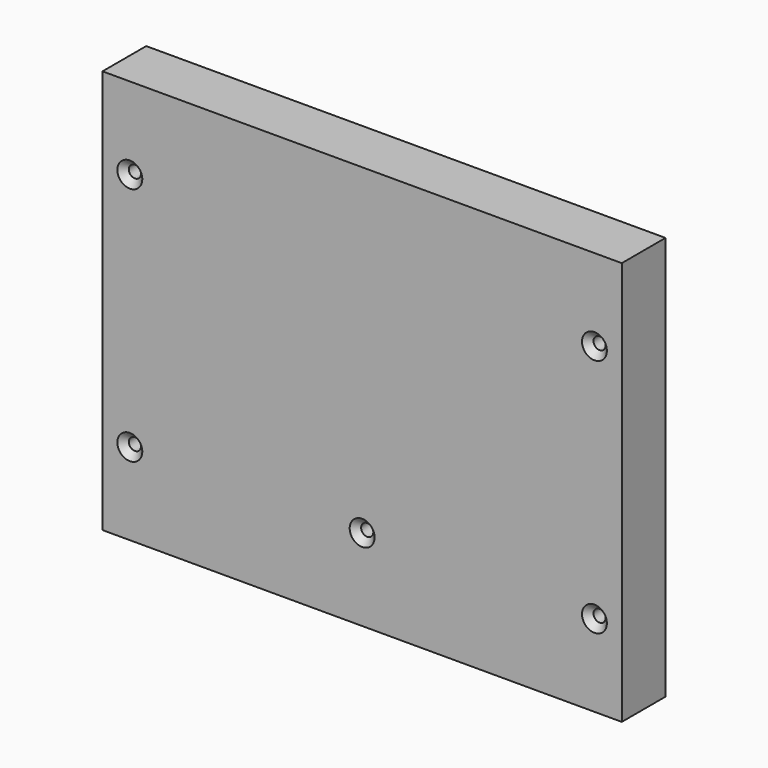
from build123d import *

# Parameters (mm, degrees)
F0_W           = 171
F0_H           = 133
F1_DEPTH       = 18
F4_D           = 4
F4_CSINK_D     = 8.2
F4_CSINK_ANGLE = 90
F5_D           = 4
F5_CSINK_D     = 8.2
F5_CSINK_ANGLE = 90
F7_D           = 4
F7_CSINK_D     = 8.2
F7_CSINK_ANGLE = 90


# Not quite as in the source:
# - a feature of the source that left no trace in its solid (it failed there, or was rolled back) is left out


with BuildPart() as f1:
    # F0 (on Front) → F1 (new body)
    with BuildSketch(Plane.XZ):
        Rectangle(F0_W, F0_H)
    extrude(amount=F1_DEPTH)

    # F4 (through all)
    with Locations(Plane.XZ.offset(18)):
        with Locations((0, -39.5)):
            CounterSinkHole(F4_D / 2, F4_CSINK_D / 2, counter_sink_angle=F4_CSINK_ANGLE)

    # F5 (through all)
    with Locations(Plane.XZ.offset(18)):
        with Locations((-76.5, -39.5), (76.5, -39.5)):
            CounterSinkHole(F5_D / 2, F5_CSINK_D / 2, counter_sink_angle=F5_CSINK_ANGLE)

    # F7 (through all)
    with Locations(Plane.XZ.offset(18)):
        with Locations((-76.5, 39.5), (76.5, 39.5)):
            CounterSinkHole(F7_D / 2, F7_CSINK_D / 2, counter_sink_angle=F7_CSINK_ANGLE)


solid = f1.part
